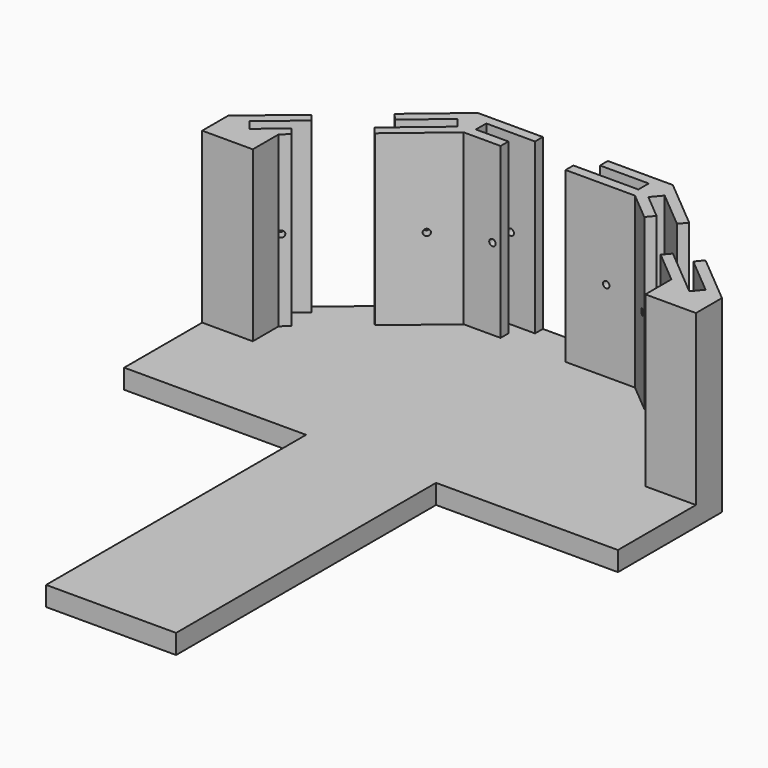
from build123d import *

# Parameters (mm, degrees)
F1_DEPTH  = 36.83
F3_DEPTH  = 33.02
F5_DEPTH  = 33.02
F6_R      = 0.635
F7_DEPTH  = 6.35
F9_R      = 0.635
F10_DEPTH = 6.35
F8_R      = 0.635
F11_DEPTH = 6.35
F12_W     = 25.4
F12_H     = 63.5
F13_DEPTH = 3.81


with BuildPart() as f1:
    # F0 (on Top) → F1 (new body)
    with BuildSketch(Plane.XY):
        Polygon((-19.05, 24.4902079291), (-48.2362932828, 0), (-48.2362932828, -25.4), (48.2362932828, -25.4), (48.2362932828, 0), (19.05, 24.4902079291), align=None)
    extrude(amount=F1_DEPTH)

    # F2 (on face) → F3 (cut)
    with BuildSketch(Plane.XY.offset(36.83)):
        Polygon((-16.7387890124, 18.1402079291), (-38.3574469823, 0), (-38.3574469823, -6.35), (-48.2362932828, -6.35), (-48.2362932828, -25.4), (-38.3574469823, -25.4), (38.3574469823, -25.4), (48.2362932828, -25.4), (48.2362932828, -6.35), (38.3574469823, -6.35), (38.3574469823, 0), (16.7387890124, 18.1402079291), align=None)
    extrude(amount=-F3_DEPTH, mode=Mode.SUBTRACT)

    # F4 (on face) → F5 (cut)
    with BuildSketch(Plane.XY.offset(36.83)):
        Polygon((15.875, 22.5852079291), (6.35, 22.5852079291), (6.35, 24.4902079291), (-6.35, 24.4902079291), (-6.35, 22.5852079291), (-15.875, 22.5852079291), (-15.875, 20.0452079291), (-9.525, 20.0452079291), (-9.525, 18.1402079291), (3.175, 18.1402079291), (3.175, 20.0452079291), (15.875, 20.0452079291), align=None)
        Polygon((22.2648719992, 13.503273733), (31.9936364268, 5.33987109), (33.2181468233, 6.7991857541), (42.9469112509, -1.3642168889), (44.5795917795, 0.5815359966), (37.2830184588, 6.7040879789), (38.5075288552, 8.163402643), (28.7787644276, 16.326805286), (27.5542540312, 14.8674906219), (20.2576807104, 20.9900426042), (18.6250001818, 19.0442897186), (23.4893823957, 14.9625883971), align=None)
        Polygon((-42.9469112509, -1.3642168889), (-38.0825290371, 2.7174844326), (-36.8580186406, 1.2581697685), (-27.129254213, 9.4215724115), (-28.3537646095, 10.8808870756), (-18.6250001818, 19.0442897186), (-20.2576807104, 20.9900426042), (-27.5542540312, 14.8674906219), (-28.7787644276, 16.326805286), (-38.5075288552, 8.163402643), (-37.2830184588, 6.7040879789), (-44.5795917795, 0.5815359966), align=None)
    extrude(amount=-F5_DEPTH, mode=Mode.SUBTRACT)

    # F6 (on face) → F7 (cut, through all)
    with BuildSketch(Plane(origin=(-19.9300744284, 23.7517378008, 0), x_dir=(-0.7660444431, -0.6427876097, 0), z_dir=(-0.6427876097, 0.7660444431, 0))):
        with Locations((6.788644426, 19.685)):
            Circle(F6_R)
        with Locations((29.013644426, 19.685)):
            Circle(F6_R)
    extrude(amount=-F7_DEPTH, mode=Mode.SUBTRACT)

    # F9 (on face) → F10 (cut, through all)
    with BuildSketch(Plane(origin=(19.9300744284, 23.7517378008, 0), x_dir=(-0.7660444431, 0.6427876097, 0), z_dir=(0.6427876097, 0.7660444431, 0))):
        with Locations((-29.013644426, 19.685)):
            Circle(F9_R)
        with Locations((-6.788644426, 19.685)):
            Circle(F9_R)
    extrude(amount=-F10_DEPTH, mode=Mode.SUBTRACT)

    # F8 (on face) → F11 (cut, through all)
    with BuildSketch(Plane(origin=(0, 24.4902079291, 0), x_dir=(-1, 0, 0), z_dir=(0, 1, 0))):
        with Locations((-11.1125, 19.685)):
            Circle(F8_R)
        with Locations((11.1125, 19.685)):
            Circle(F8_R)
    extrude(amount=-F11_DEPTH, mode=Mode.SUBTRACT)

    # F12 (on face) → F13 (join, through all)
    with BuildSketch(Plane(origin=(0, 0, 0), x_dir=(1, 0, 0), z_dir=(0, 0, -1))):
        with Locations((0, 57.15)):
            Rectangle(F12_W, F12_H)
    extrude(amount=-F13_DEPTH)


solid = f1.part
